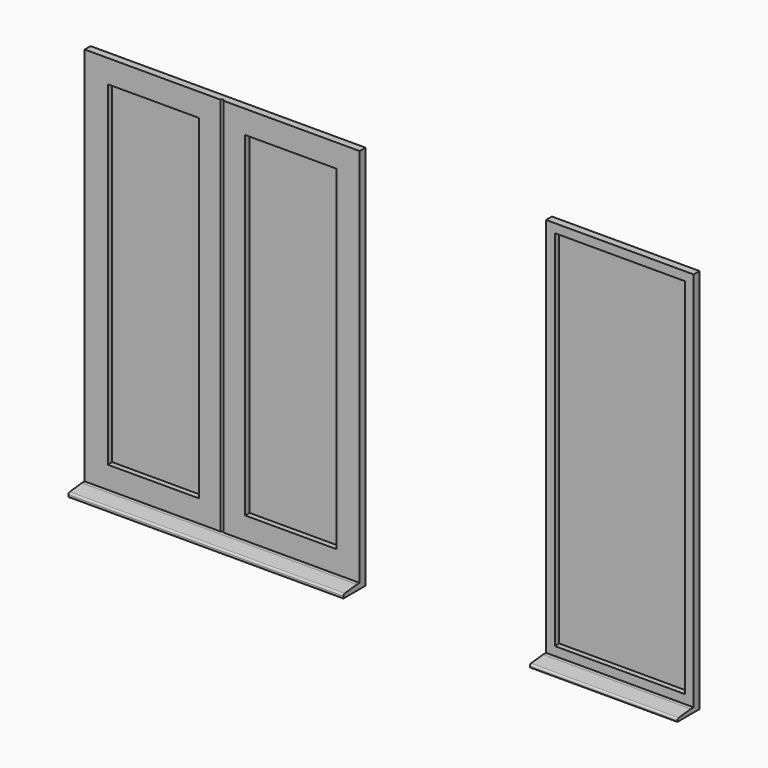
from build123d import *

# Parameters (mm, degrees)
F1_W      = 150
F1_H      = 30
F2_DEPTH  = 1490
F3_SIZE2  = 90
F3_SIZE   = 10
F4_R      = 10
F0_W      = 745
F0_H      = 2065
F0_W_2    = 495
F0_H_2    = 1815
F5_DEPTH  = 40
F6_SIZE   = 8
F7_DEPTH  = 40
F8_SIZE   = 7.99999
F9_DEPTH  = 10
F10_DEPTH = 10
F13_W     = 150
F13_H     = 25
F14_DEPTH = 800
F15_SIZE2 = 90
F15_SIZE  = 10
F16_R     = 10
F12_W     = 800
F12_H     = 2065
F12_W_2   = 705
F12_H_2   = 1970
F17_DEPTH = 40
F18_DEPTH = 10


# Not quite as in the source:
# - a fillet or chamfer is up to 0.001 mm smaller than in the source, because OpenCascade refuses the exact size


with BuildPart() as f2:
    # F1 (on Right) → F2 (new body)
    with BuildSketch(Plane.YZ):
        with Locations((-75, 15)):
            Rectangle(F1_W, F1_H)
    extrude(amount=F2_DEPTH)

    # F3
    f3_edges = [f2.edges().sort_by_distance(p)[0] for p in [
        (745, -150, 30),
    ]]
    f3_side = f2.faces().sort_by_distance((745, -150, 15))[0]
    chamfer(f3_edges, length=F3_SIZE, length2=F3_SIZE2, reference=f3_side)

    # F4
    f4_edges = [f2.edges().sort_by_distance(p)[0] for p in [
        (745, -150, 20),
    ]]
    fillet(f4_edges, radius=F4_R)

    # F0 (on Front) → F5 (join)
    with BuildSketch(Plane.XZ):
        with Locations((372.5, 1057.5)):
            Rectangle(F0_W, F0_H)
        with Locations((372.5, 1057.5)):
            Rectangle(F0_W_2, F0_H_2, mode=Mode.SUBTRACT)
    extrude(amount=F5_DEPTH)

    # F6
    f6_edges = [f2.edges().sort_by_distance(p)[0] for p in [
        (745, -40, 1060),
    ]]
    chamfer(f6_edges, length=F6_SIZE)

    # F0 (on Front) → F7 (join)
    with BuildSketch(Plane.XZ):
        with Locations((1117.5, 1057.5)):
            Rectangle(F0_W, F0_H)
        with Locations((1117.5, 1057.5)):
            Rectangle(F0_W_2, F0_H_2, mode=Mode.SUBTRACT)
    extrude(amount=F7_DEPTH)

    # F8 (size 8 in the source; OpenCascade refuses exactly that, so slightly less here)
    f8_edges = [f2.edges().sort_by_distance(p)[0] for p in [
        (745, -40, 1060),
    ]]
    chamfer(f8_edges, length=F8_SIZE)


with BuildPart() as f9:
    # F0 (on Front) → F9 (new body)
    with BuildSketch(Plane.XZ):
        with Locations((372.5, 1057.5)):
            Rectangle(F0_W_2, F0_H_2)
    extrude(amount=F9_DEPTH)


with BuildPart() as f10:
    # F0 (on Front) → F10 (new body)
    with BuildSketch(Plane.XZ):
        with Locations((1117.5, 1057.5)):
            Rectangle(F0_W_2, F0_H_2)
    extrude(amount=F10_DEPTH)


with BuildPart() as f14:
    # F13 (on offset) → F14 (new body)
    with BuildSketch(Plane.YZ.offset(2500)):
        with Locations((-75, 12.5)):
            Rectangle(F13_W, F13_H)
    extrude(amount=F14_DEPTH)

    # F15
    f15_edges = [f14.edges().sort_by_distance(p)[0] for p in [
        (2900, -150, 25),
    ]]
    f15_side = f14.faces().sort_by_distance((2900, -150, 12.5))[0]
    chamfer(f15_edges, length=F15_SIZE, length2=F15_SIZE2, reference=f15_side)

    # F16
    f16_edges = [f14.edges().sort_by_distance(p)[0] for p in [
        (2900, -150, 15),
    ]]
    fillet(f16_edges, radius=F16_R)

    # F12 (on Front) → F17 (join)
    with BuildSketch(Plane.XZ):
        with Locations((2900, 1057.5)):
            Rectangle(F12_W, F12_H)
        with Locations((2900, 1057.5)):
            Rectangle(F12_W_2, F12_H_2, mode=Mode.SUBTRACT)
    extrude(amount=F17_DEPTH)


with BuildPart() as f18:
    # F12 (on Front) → F18 (new body)
    with BuildSketch(Plane.XZ):
        with Locations((2900, 1057.5)):
            Rectangle(F12_W_2, F12_H_2)
    extrude(amount=F18_DEPTH)


solid = Compound([f2.part, f9.part, f10.part, f14.part, f18.part])
